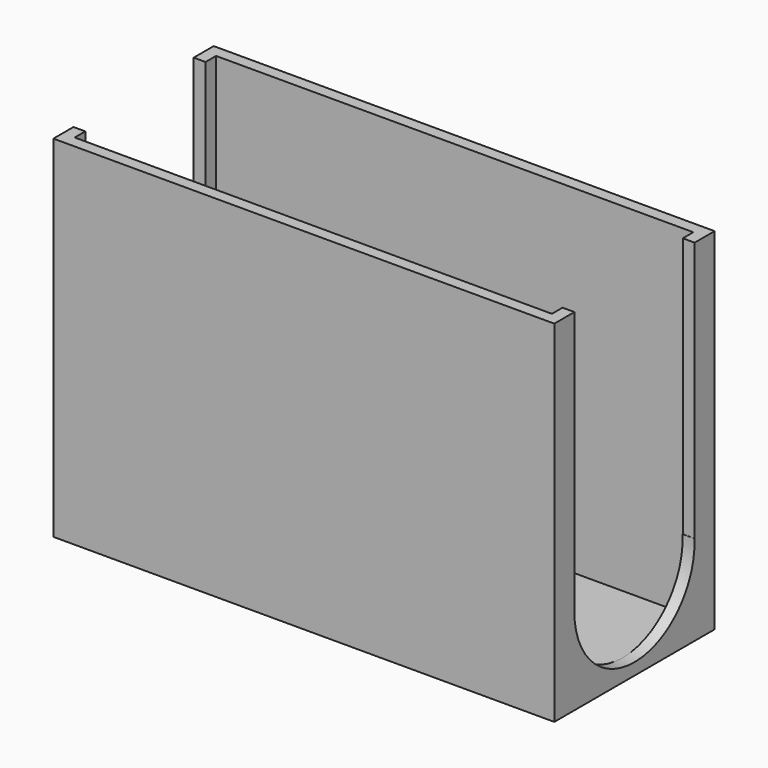
from build123d import *

# Parameters (mm, degrees)
F0_W     = 63.5
F0_H     = 25.4
F1_DEPTH = 44.45
F2_T     = -1.5
F4_DEPTH = 1.5


# Not quite as in the source:
# - a pattern or mirror of a feature is missing from the dataset's text; its kind, count and spacing are read off the source's solid


with BuildPart() as f1:
    # F0 (on Top) → F1 (new body)
    with BuildSketch(Plane.XY):
        Rectangle(F0_W, F0_H)
    extrude(amount=F1_DEPTH)

    # F2
    f2_openings = [f1.faces().sort_by_distance(p)[0] for p in [
        (0, 0, 44.45),
    ]]
    offset(amount=F2_T, openings=f2_openings)

    # F3 (on face) → F4 (cut)
    with BuildSketch(Plane(origin=(-31.75, 0, 0), x_dir=(0, -1, 0), z_dir=(-1, 0, 0))):
        with BuildLine():
            Line((-9.5163858686, 11.43), (9.5163858686, 11.43))
            ThreePointArc((9.5163858686, 11.43), (0, 20.55), (-9.5163858686, 11.43))
        make_face()
        with BuildLine():
            ThreePointArc((-9.5163858686, 11.43), (-0.2025457993, 1.5021537764), (9.525, 11.025))
            ThreePointArc((9.525, 11.025), (9.5228462236, 11.2275457993), (9.5163858686, 11.43))
            Line((9.5163858686, 11.43), (-9.5163858686, 11.43))
        make_face()
        with BuildLine():
            ThreePointArc((-9.5163858686, 11.43), (0, 20.55), (9.5163858686, 11.43))
            Line((9.5163858686, 11.43), (9.5163858686, 44.45))
            Line((9.5163858686, 44.45), (-9.5336141314, 44.45))
            Line((-9.5336141314, 44.45), (-9.5336141314, 11.43))
            Line((-9.5336141314, 11.43), (-9.5163858686, 11.43))
        make_face()
    f4 = extrude(amount=-F4_DEPTH, mode=Mode.SUBTRACT)

    # F4_copies: F4 across plane
    add(f4.mirror(Plane(origin=(0, 0, 0), x_dir=(0, 0, 1), z_dir=(1, 0, 0))), mode=Mode.SUBTRACT)


solid = f1.part
